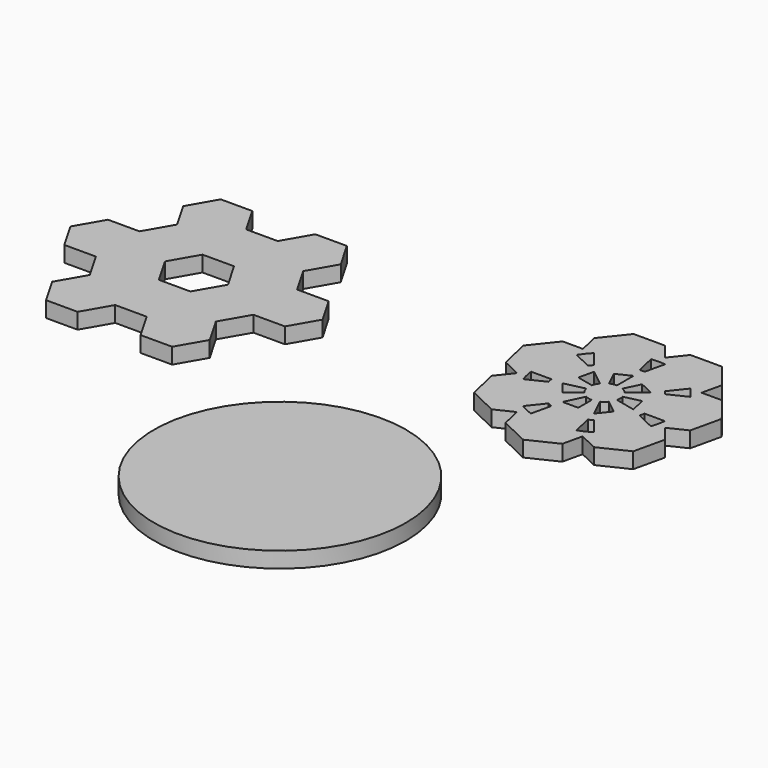
from build123d import *

# Parameters (mm, degrees)
F1_DEPTH = 5
F0_R     = 40


with BuildPart() as f1:
    # F0 (on Top) → F1 (new body)
    with BuildSketch(Plane.XY):
        Polygon((-6.3519277994, -7.4067961433), (-11.3519277994, 1.2534578946), (-21.3519277994, 1.2534578946), (-26.3519277994, -7.4067961433), (-21.3519277994, -16.0670501811), (-11.3519277994, -16.0670501811), align=None)
        Polygon((-6.3519277994, 9.9137119324), (-11.3519277994, 1.2534578946), (-6.3519277994, -7.4067961433), (3.6480722006, -7.4067961433), (8.6480722006, 1.2534578946), (3.6480722006, 9.9137119324), align=None)
        Polygon((-26.3519277994, -7.4067961433), (-21.3519277994, 1.2534578946), (-26.3519277994, 9.9137119324), (-36.3519277994, 9.9137119324), (-41.3519277994, 1.2534578946), (-36.3519277994, -7.4067961433), align=None)
        Polygon((-11.3519277994, 18.5739659703), (-6.3519277994, 9.9137119324), (3.6480722006, 9.9137119324), (8.6480722006, 18.5739659703), (3.6480722006, 27.2342200081), (-6.3519277994, 27.2342200081), align=None)
        Polygon((3.6480722006, -7.4067961433), (-6.3519277994, -7.4067961433), (-11.3519277994, -16.0670501811), (-6.3519277994, -24.727304219), (3.6480722006, -24.727304219), (8.6480722006, -16.0670501811), align=None)
        Polygon((-36.3519277994, 9.9137119324), (-26.3519277994, 9.9137119324), (-21.3519277994, 18.5739659703), (-26.3519277994, 27.2342200081), (-36.3519277994, 27.2342200081), (-41.3519277994, 18.5739659703), align=None)
        Polygon((-21.3519277994, -16.0670501811), (-26.3519277994, -7.4067961433), (-36.3519277994, -7.4067961433), (-41.3519277994, -16.0670501811), (-36.3519277994, -24.727304219), (-26.3519277994, -24.727304219), align=None)
        Polygon((-21.3519277994, 18.5739659703), (-11.3519277994, 18.5739659703), (-6.3519277994, 27.2342200081), (-11.3519277994, 35.894474046), (-21.3519277994, 35.894474046), (-26.3519277994, 27.2342200081), align=None)
        Polygon((8.6480722006, 18.5739659703), (3.6480722006, 9.9137119324), (8.6480722006, 1.2534578946), (18.6480722006, 1.2534578946), (23.6480722006, 9.9137119324), (18.6480722006, 18.5739659703), align=None)
        Polygon((-41.3519277994, 1.2534578946), (-36.3519277994, 9.9137119324), (-41.3519277994, 18.5739659703), (-51.3519277994, 18.5739659703), (-56.3519277994, 9.9137119324), (-51.3519277994, 1.2534578946), align=None)
        Polygon((-11.3519277994, 35.894474046), (-6.3519277994, 27.2342200081), (3.6480722006, 27.2342200081), (8.6480722006, 35.894474046), (3.6480722006, 44.5547280838), (-6.3519277994, 44.5547280838), align=None)
        Polygon((-36.3519277994, 27.2342200081), (-26.3519277994, 27.2342200081), (-21.3519277994, 35.894474046), (-26.3519277994, 44.5547280838), (-36.3519277994, 44.5547280838), (-41.3519277994, 35.894474046), align=None)
    extrude(amount=F1_DEPTH)


with BuildPart() as f1b:
    # F0 (on Top) → F1, piece 2 (new body)
    with BuildSketch(Plane.XY):
        with BuildLine():
            Line((108.4534161646, 9.1103293915), (107.6647373891, 12.5657568802))
            Line((107.6647373891, 12.5657568802), (102.6647373891, 12.5657568802))
            Line((102.6647373891, 12.5657568802), (97.6647373891, 12.5657568802))
            Line((97.6647373891, 12.5657568802), (96.8760586136, 9.1103293915))
            ThreePointArc((96.8760586136, 9.1103293915), (102.6647373891, 7.948363863), (108.4534161646, 9.1103293915))
        make_face()
        with BuildLine():
            Line((109.8745662116, 9.7947191837), (107.6647373891, 12.5657568802))
            Line((107.6647373891, 12.5657568802), (108.4534161646, 9.1103293915))
            ThreePointArc((108.4534161646, 9.1103293915), (109.1729934758, 9.4338308445), (109.8745662116, 9.7947191837))
        make_face()
        with BuildLine():
            Line((110.7821863984, 16.4749142925), (107.6647373891, 12.5657568802))
            Line((107.6647373891, 12.5657568802), (109.8745662116, 9.7947191837))
            ThreePointArc((109.8745662116, 9.7947191837), (114.3922096261, 13.5960168351), (117.0929305771, 18.8462618009))
            Line((117.0929305771, 18.8462618009), (113.8996354077, 20.3840717048))
            Line((113.8996354077, 20.3840717048), (110.7821863984, 16.4749142925))
        make_face()
        with BuildLine():
            Line((102.6647373891, 12.5657568802), (107.6647373891, 12.5657568802))
            Line((107.6647373891, 12.5657568802), (104.8341560847, 18.4435195235))
            ThreePointArc((104.8341560847, 18.4435195235), (103.7773420588, 18.0737243021), (102.6647373891, 17.948363863))
            Line((102.6647373891, 17.948363863), (102.6647373891, 12.5657568802))
        make_face()
        with BuildLine():
            Line((106.5738948014, 19.8309148537), (110.7821863984, 16.4749142925))
            Line((110.7821863984, 16.4749142925), (113.8996354077, 20.3840717048))
            Line((113.8996354077, 20.3840717048), (107.53937695, 21.8357591932))
            ThreePointArc((107.53937695, 21.8357591932), (107.1695817286, 20.7789451674), (106.5738948014, 19.8309148537))
        make_face()
        with BuildLine():
            Line((109.8899467286, 2.8164777583), (108.4534161646, 9.1103293915))
            ThreePointArc((108.4534161646, 9.1103293915), (102.6647373891, 7.948363863), (96.8760586136, 9.1103293915))
            Line((96.8760586136, 9.1103293915), (95.4395280495, 2.8164777583))
            ThreePointArc((95.4395280495, 2.8164777583), (102.6647373891, 1.5591963212), (109.8899467286, 2.8164777583))
        make_face()
        with BuildLine():
            ThreePointArc((117.0929305771, 18.8462618009), (114.3922096261, 13.5960168351), (109.8745662116, 9.7947191837))
            Line((109.8745662116, 9.7947191837), (113.8996354077, 4.7474420555))
            ThreePointArc((113.8996354077, 4.7474420555), (119.3874619571, 9.6124360304), (122.9093240867, 16.0452343137))
            Line((122.9093240867, 16.0452343137), (117.0929305771, 18.8462618009))
        make_face()
        with BuildLine():
            ThreePointArc((102.6647373891, 17.948363863), (103.7773420588, 18.0737243021), (104.8341560847, 18.4435195235))
            Line((104.8341560847, 18.4435195235), (102.6647373891, 22.948363863))
            Line((102.6647373891, 22.948363863), (102.6647373891, 17.948363863))
        make_face()
        with BuildLine():
            Line((102.6647373891, 22.948363863), (104.8341560847, 18.4435195235))
            ThreePointArc((104.8341560847, 18.4435195235), (105.7821863984, 19.0392064507), (106.5738948014, 19.8309148537))
            Line((106.5738948014, 19.8309148537), (102.6647373891, 22.948363863))
        make_face()
        with BuildLine():
            Line((95.4549085665, 9.7947191837), (97.6647373891, 12.5657568802))
            Line((97.6647373891, 12.5657568802), (94.5472883798, 16.4749142925))
            Line((94.5472883798, 16.4749142925), (91.4298393705, 20.3840717048))
            Line((91.4298393705, 20.3840717048), (88.236544201, 18.8462618009))
            ThreePointArc((88.236544201, 18.8462618009), (90.937265152, 13.5960168351), (95.4549085665, 9.7947191837))
        make_face()
        with BuildLine():
            Line((96.8760586136, 9.1103293915), (97.6647373891, 12.5657568802))
            Line((97.6647373891, 12.5657568802), (95.4549085665, 9.7947191837))
            ThreePointArc((95.4549085665, 9.7947191837), (96.1564813023, 9.4338308445), (96.8760586136, 9.1103293915))
        make_face()
        with BuildLine():
            Line((94.5472883798, 16.4749142925), (97.6647373891, 12.5657568802))
            Line((97.6647373891, 12.5657568802), (100.4953186935, 18.4435195235))
            ThreePointArc((100.4953186935, 18.4435195235), (99.5472883798, 19.0392064507), (98.7555799767, 19.8309148537))
            Line((98.7555799767, 19.8309148537), (94.5472883798, 16.4749142925))
        make_face()
        with BuildLine():
            ThreePointArc((100.4953186935, 18.4435195235), (101.5521327193, 18.0737243021), (102.6647373891, 17.948363863))
            Line((102.6647373891, 17.948363863), (102.6647373891, 22.948363863))
            Line((102.6647373891, 22.948363863), (100.4953186935, 18.4435195235))
        make_face()
        with BuildLine():
            Line((117.4439256526, 20.3840717048), (113.8996354077, 20.3840717048))
            Line((113.8996354077, 20.3840717048), (117.0929305771, 18.8462618009))
            ThreePointArc((117.0929305771, 18.8462618009), (117.2886560718, 19.6105498537), (117.4439256526, 20.3840717048))
        make_face()
        with BuildLine():
            Line((112.7870307379, 25.2587112658), (113.8996354077, 20.3840717048))
            Line((113.8996354077, 20.3840717048), (117.4439256526, 20.3840717048))
            ThreePointArc((117.4439256526, 20.3840717048), (117.6094325006, 21.661473027), (117.6647373891, 22.948363863))
            ThreePointArc((117.6647373891, 22.948363863), (116.9483776416, 27.5284971729), (114.8677212376, 31.6711607306))
            Line((114.8677212376, 31.6711607306), (111.6744260681, 30.1333508267))
            Line((111.6744260681, 30.1333508267), (112.7870307379, 25.2587112658))
        make_face()
        with BuildLine():
            Line((102.6647373891, 22.948363863), (106.5738948014, 19.8309148537))
            ThreePointArc((106.5738948014, 19.8309148537), (107.1695817286, 20.7789451674), (107.53937695, 21.8357591932))
            Line((107.53937695, 21.8357591932), (102.6647373891, 22.948363863))
        make_face()
        with BuildLine():
            ThreePointArc((113.8996354077, 4.7474420555), (111.9451493787, 3.6773897975), (109.8899467286, 2.8164777583))
            Line((109.8899467286, 2.8164777583), (113.1054673892, 1.267964622))
            Line((113.1054673892, 1.267964622), (113.8996354077, 4.7474420555))
        make_face()
        with BuildLine():
            Line((113.1054673892, 1.267964622), (109.8899467286, 2.8164777583))
            ThreePointArc((109.8899467286, 2.8164777583), (102.6647373891, 1.5591963212), (95.4395280495, 2.8164777583))
            Line((95.4395280495, 2.8164777583), (92.224007389, 1.267964622))
            Line((92.224007389, 1.267964622), (93.65504871, -5.0018370663))
            ThreePointArc((93.65504871, -5.0018370663), (102.6647373891, -6.4180833529), (111.6744260681, -5.0018370663))
            Line((111.6744260681, -5.0018370663), (113.1054673892, 1.267964622))
        make_face()
        with BuildLine():
            ThreePointArc((122.9093240867, 16.0452343137), (119.3874619571, 9.6124360304), (113.8996354077, 4.7474420555))
            Line((113.8996354077, 4.7474420555), (113.1054673892, 1.267964622))
            Line((113.1054673892, 1.267964622), (118.8996354077, -1.5223596328))
            ThreePointArc((118.8996354077, -1.5223596328), (125.6243503507, 4.6386835071), (130.1345334262, 12.5657568802))
            Line((130.1345334262, 12.5657568802), (126.1248447472, 17.59374745))
            Line((126.1248447472, 17.59374745), (122.9093240867, 16.0452343137))
        make_face()
        with BuildLine():
            Line((97.7900978282, 24.0609685328), (102.6647373891, 22.948363863))
            Line((102.6647373891, 22.948363863), (98.7555799767, 26.0658128723))
            ThreePointArc((98.7555799767, 26.0658128723), (98.1598930496, 25.1177825586), (97.7900978282, 24.0609685328))
        make_face()
        with BuildLine():
            Line((98.7555799767, 26.0658128723), (102.6647373891, 22.948363863))
            Line((102.6647373891, 22.948363863), (100.4953186935, 27.4532082025))
            ThreePointArc((100.4953186935, 27.4532082025), (99.5472883798, 26.8575212754), (98.7555799767, 26.0658128723))
        make_face()
        with BuildLine():
            Line((98.7555799767, 19.8309148537), (102.6647373891, 22.948363863))
            Line((102.6647373891, 22.948363863), (97.7900978282, 21.8357591932))
            ThreePointArc((97.7900978282, 21.8357591932), (98.1598930496, 20.7789451674), (98.7555799767, 19.8309148537))
        make_face()
        with BuildLine():
            Line((106.5738948014, 26.0658128723), (102.6647373891, 22.948363863))
            Line((102.6647373891, 22.948363863), (107.53937695, 24.0609685328))
            ThreePointArc((107.53937695, 24.0609685328), (107.1695817286, 25.1177825586), (106.5738948014, 26.0658128723))
        make_face()
        with BuildLine():
            Line((102.6647373891, 27.948363863), (102.6647373891, 22.948363863))
            Line((102.6647373891, 22.948363863), (104.8341560847, 27.4532082025))
            ThreePointArc((104.8341560847, 27.4532082025), (103.7773420588, 27.8230034239), (102.6647373891, 27.948363863))
        make_face()
        with BuildLine():
            Line((104.8341560847, 27.4532082025), (102.6647373891, 22.948363863))
            Line((102.6647373891, 22.948363863), (106.5738948014, 26.0658128723))
            ThreePointArc((106.5738948014, 26.0658128723), (105.7821863984, 26.8575212754), (104.8341560847, 27.4532082025))
        make_face()
        with BuildLine():
            Line((100.4953186935, 18.4435195235), (102.6647373891, 22.948363863))
            Line((102.6647373891, 22.948363863), (98.7555799767, 19.8309148537))
            ThreePointArc((98.7555799767, 19.8309148537), (99.5472883798, 19.0392064507), (100.4953186935, 18.4435195235))
        make_face()
        with BuildLine():
            Line((107.53937695, 24.0609685328), (102.6647373891, 22.948363863))
            Line((102.6647373891, 22.948363863), (107.53937695, 21.8357591932))
            ThreePointArc((107.53937695, 21.8357591932), (107.6332984385, 22.3885414825), (107.6647373891, 22.948363863))
            ThreePointArc((107.6647373891, 22.948363863), (107.6332984385, 23.5081862435), (107.53937695, 24.0609685328))
        make_face()
        with BuildLine():
            Line((97.7900978282, 21.8357591932), (102.6647373891, 22.948363863))
            Line((102.6647373891, 22.948363863), (97.7900978282, 24.0609685328))
            ThreePointArc((97.7900978282, 24.0609685328), (97.6647373891, 22.948363863), (97.7900978282, 21.8357591932))
        make_face()
        with BuildLine():
            Line((100.4953186935, 27.4532082025), (102.6647373891, 22.948363863))
            Line((102.6647373891, 22.948363863), (102.6647373891, 27.948363863))
            ThreePointArc((102.6647373891, 27.948363863), (101.5521327193, 27.8230034239), (100.4953186935, 27.4532082025))
        make_face()
        with BuildLine():
            Line((91.4298393705, 4.7474420555), (95.4549085665, 9.7947191837))
            ThreePointArc((95.4549085665, 9.7947191837), (90.937265152, 13.5960168351), (88.236544201, 18.8462618009))
            Line((88.236544201, 18.8462618009), (82.4201506915, 16.0452343137))
            ThreePointArc((82.4201506915, 16.0452343137), (85.9420128211, 9.6124360304), (91.4298393705, 4.7474420555))
        make_face()
        with BuildLine():
            Line((107.53937695, 24.0609685328), (112.7870307379, 25.2587112658))
            Line((112.7870307379, 25.2587112658), (111.6744260681, 30.1333508267))
            Line((111.6744260681, 30.1333508267), (106.5738948014, 26.0658128723))
            ThreePointArc((106.5738948014, 26.0658128723), (107.1695817286, 25.1177825586), (107.53937695, 24.0609685328))
        make_face()
        with BuildLine():
            ThreePointArc((117.6647373891, 22.948363863), (117.6094325006, 21.661473027), (117.4439256526, 20.3840717048))
            Line((117.4439256526, 20.3840717048), (123.8996354077, 20.3840717048))
            ThreePointArc((123.8996354077, 20.3840717048), (124.0153027163, 21.6638996403), (124.0539049309, 22.948363863))
            ThreePointArc((124.0539049309, 22.948363863), (123.194179289, 28.9515716231), (120.6841147471, 34.4721882178))
            Line((120.6841147471, 34.4721882178), (114.8677212376, 31.6711607306))
            ThreePointArc((114.8677212376, 31.6711607306), (116.9483776416, 27.5284971729), (117.6647373891, 22.948363863))
        make_face()
        with BuildLine():
            Line((92.224007389, 1.267964622), (95.4395280495, 2.8164777583))
            ThreePointArc((95.4395280495, 2.8164777583), (93.3843253994, 3.6773897975), (91.4298393705, 4.7474420555))
            Line((91.4298393705, 4.7474420555), (92.224007389, 1.267964622))
        make_face()
        with BuildLine():
            ThreePointArc((123.8996354077, 20.3840717048), (123.5176338439, 18.1888263251), (122.9093240867, 16.0452343137))
            Line((122.9093240867, 16.0452343137), (126.1248447472, 17.59374745))
            Line((126.1248447472, 17.59374745), (123.8996354077, 20.3840717048))
        make_face()
        with BuildLine():
            Line((93.65504871, 30.1333508267), (98.7555799767, 26.0658128723))
            ThreePointArc((98.7555799767, 26.0658128723), (99.5472883798, 26.8575212754), (100.4953186935, 27.4532082025))
            Line((100.4953186935, 27.4532082025), (98.1598930496, 32.3027695223))
            Line((98.1598930496, 32.3027695223), (93.65504871, 30.1333508267))
        make_face()
        with BuildLine():
            Line((91.4298393705, 20.3840717048), (97.7900978282, 21.8357591932))
            ThreePointArc((97.7900978282, 21.8357591932), (97.6647373891, 22.948363863), (97.7900978282, 24.0609685328))
            Line((97.7900978282, 24.0609685328), (92.5424440403, 25.2587112658))
            Line((92.5424440403, 25.2587112658), (91.4298393705, 20.3840717048))
        make_face()
        with BuildLine():
            ThreePointArc((102.6647373891, 27.948363863), (103.7773420588, 27.8230034239), (104.8341560847, 27.4532082025))
            Line((104.8341560847, 27.4532082025), (107.1695817286, 32.3027695223))
            Line((107.1695817286, 32.3027695223), (102.6647373891, 34.4721882178))
            Line((102.6647373891, 34.4721882178), (102.6647373891, 27.948363863))
        make_face()
        with BuildLine():
            Line((87.8855491256, 20.3840717048), (91.4298393705, 20.3840717048))
            Line((91.4298393705, 20.3840717048), (92.5424440403, 25.2587112658))
            Line((92.5424440403, 25.2587112658), (93.65504871, 30.1333508267))
            Line((93.65504871, 30.1333508267), (90.4617535406, 31.6711607306))
            ThreePointArc((90.4617535406, 31.6711607306), (88.0408187063, 26.2861778724), (87.8855491256, 20.3840717048))
        make_face()
        with BuildLine():
            Line((88.236544201, 18.8462618009), (91.4298393705, 20.3840717048))
            Line((91.4298393705, 20.3840717048), (87.8855491256, 20.3840717048))
            ThreePointArc((87.8855491256, 20.3840717048), (88.0408187063, 19.6105498537), (88.236544201, 18.8462618009))
        make_face()
        with BuildLine():
            Line((92.224007389, 1.267964622), (91.4298393705, 4.7474420555))
            ThreePointArc((91.4298393705, 4.7474420555), (85.9420128211, 9.6124360304), (82.4201506915, 16.0452343137))
            Line((82.4201506915, 16.0452343137), (79.2046300309, 17.59374745))
            Line((79.2046300309, 17.59374745), (75.1949413519, 12.5657568802))
            ThreePointArc((75.1949413519, 12.5657568802), (79.7051244274, 4.6386835071), (86.4298393705, -1.5223596328))
            Line((86.4298393705, -1.5223596328), (92.224007389, 1.267964622))
        make_face()
        with BuildLine():
            Line((113.8842548906, 32.9043885231), (111.6744260681, 30.1333508267))
            Line((111.6744260681, 30.1333508267), (114.8677212376, 31.6711607306))
            ThreePointArc((114.8677212376, 31.6711607306), (114.3922096261, 32.3007108909), (113.8842548906, 32.9043885231))
        make_face()
        with BuildLine():
            Line((107.1695817286, 32.3027695223), (111.6744260681, 30.1333508267))
            Line((111.6744260681, 30.1333508267), (113.8842548906, 32.9043885231))
            ThreePointArc((113.8842548906, 32.9043885231), (109.1729934758, 36.4628968816), (103.4534161646, 37.9276157065))
            Line((103.4534161646, 37.9276157065), (102.6647373891, 34.4721882178))
            Line((102.6647373891, 34.4721882178), (107.1695817286, 32.3027695223))
        make_face()
        with BuildLine():
            ThreePointArc((124.0539049309, 22.948363863), (124.0153027163, 21.6638996403), (123.8996354077, 20.3840717048))
            Line((123.8996354077, 20.3840717048), (126.1248447472, 17.59374745))
            Line((126.1248447472, 17.59374745), (131.9190127657, 20.3840717048))
            ThreePointArc((131.9190127657, 20.3840717048), (132.0031282428, 21.6649916651), (132.031184605, 22.948363863))
            ThreePointArc((132.031184605, 22.948363863), (130.9819763508, 30.7279653741), (127.9093240867, 37.9516656513))
            Line((127.9093240867, 37.9516656513), (121.4782827656, 37.9516656513))
            Line((121.4782827656, 37.9516656513), (120.6841147471, 34.4721882178))
            ThreePointArc((120.6841147471, 34.4721882178), (123.194179289, 28.9515716231), (124.0539049309, 22.948363863))
        make_face()
        with BuildLine():
            ThreePointArc((130.1345334262, 12.5657568802), (125.6243503507, 4.6386835071), (118.8996354077, -1.5223596328))
            Line((118.8996354077, -1.5223596328), (127.9093240867, 2.8164777583))
            Line((127.9093240867, 2.8164777583), (130.1345334262, 12.5657568802))
        make_face()
        with BuildLine():
            Line((102.6647373891, -9.3406744575), (111.6744260681, -5.0018370663))
            ThreePointArc((111.6744260681, -5.0018370663), (102.6647373891, -6.4180833529), (93.65504871, -5.0018370663))
            Line((93.65504871, -5.0018370663), (102.6647373891, -9.3406744575))
        make_face()
        with BuildLine():
            Line((91.4452198875, 32.9043885231), (93.65504871, 30.1333508267))
            Line((93.65504871, 30.1333508267), (98.1598930496, 32.3027695223))
            Line((98.1598930496, 32.3027695223), (102.6647373891, 34.4721882178))
            Line((102.6647373891, 34.4721882178), (101.8760586136, 37.9276157065))
            ThreePointArc((101.8760586136, 37.9276157065), (96.1564813023, 36.4628968816), (91.4452198875, 32.9043885231))
        make_face()
        with BuildLine():
            Line((90.4617535406, 31.6711607306), (93.65504871, 30.1333508267))
            Line((93.65504871, 30.1333508267), (91.4452198875, 32.9043885231))
            ThreePointArc((91.4452198875, 32.9043885231), (90.937265152, 32.3007108909), (90.4617535406, 31.6711607306))
        make_face()
        with BuildLine():
            Line((101.8760586136, 37.9276157065), (102.6647373891, 34.4721882178))
            Line((102.6647373891, 34.4721882178), (103.4534161646, 37.9276157065))
            ThreePointArc((103.4534161646, 37.9276157065), (102.6647373891, 37.948363863), (101.8760586136, 37.9276157065))
        make_face()
        with BuildLine():
            Line((81.4298393705, 20.3840717048), (87.8855491256, 20.3840717048))
            ThreePointArc((87.8855491256, 20.3840717048), (88.0408187063, 26.2861778724), (90.4617535406, 31.6711607306))
            Line((90.4617535406, 31.6711607306), (84.645360031, 34.4721882178))
            ThreePointArc((84.645360031, 34.4721882178), (81.8118409342, 27.707901401), (81.4298393705, 20.3840717048))
        make_face()
        with BuildLine():
            Line((79.2046300309, 17.59374745), (82.4201506915, 16.0452343137))
            ThreePointArc((82.4201506915, 16.0452343137), (81.8118409342, 18.1888263251), (81.4298393705, 20.3840717048))
            Line((81.4298393705, 20.3840717048), (79.2046300309, 17.59374745))
        make_face()
        with BuildLine():
            ThreePointArc((103.4534161646, 37.9276157065), (109.1729934758, 36.4628968816), (113.8842548906, 32.9043885231))
            Line((113.8842548906, 32.9043885231), (117.9093240867, 37.9516656513))
            ThreePointArc((117.9093240867, 37.9516656513), (111.9451493787, 42.2193379286), (104.8899467286, 44.2214673397))
            Line((104.8899467286, 44.2214673397), (103.4534161646, 37.9276157065))
        make_face()
        with BuildLine():
            Line((77.4201506915, 2.8164777583), (86.4298393705, -1.5223596328))
            ThreePointArc((86.4298393705, -1.5223596328), (79.7051244274, 4.6386835071), (75.1949413519, 12.5657568802))
            Line((75.1949413519, 12.5657568802), (77.4201506915, 2.8164777583))
        make_face()
        with BuildLine():
            ThreePointArc((132.031184605, 22.948363863), (132.0031282428, 21.6649916651), (131.9190127657, 20.3840717048))
            Line((131.9190127657, 20.3840717048), (134.1442221053, 30.1333508267))
            Line((134.1442221053, 30.1333508267), (127.9093240867, 37.9516656513))
            ThreePointArc((127.9093240867, 37.9516656513), (130.9819763508, 30.7279653741), (132.031184605, 22.948363863))
        make_face()
        with BuildLine():
            Line((87.4201506915, 37.9516656513), (91.4452198875, 32.9043885231))
            ThreePointArc((91.4452198875, 32.9043885231), (96.1564813023, 36.4628968816), (101.8760586136, 37.9276157065))
            Line((101.8760586136, 37.9276157065), (100.4395280495, 44.2214673397))
            ThreePointArc((100.4395280495, 44.2214673397), (93.3843253994, 42.2193379286), (87.4201506915, 37.9516656513))
        make_face()
        with BuildLine():
            Line((79.2046300309, 17.59374745), (81.4298393705, 20.3840717048))
            ThreePointArc((81.4298393705, 20.3840717048), (81.8118409342, 27.707901401), (84.645360031, 34.4721882178))
            Line((84.645360031, 34.4721882178), (83.8511920125, 37.9516656513))
            Line((83.8511920125, 37.9516656513), (77.4201506915, 37.9516656513))
            ThreePointArc((77.4201506915, 37.9516656513), (74.0345683167, 29.4830131245), (73.4104620124, 20.3840717048))
            Line((73.4104620124, 20.3840717048), (79.2046300309, 17.59374745))
        make_face()
        with BuildLine():
            ThreePointArc((117.9093240867, 37.9516656513), (119.3874619571, 36.2842916956), (120.6841147471, 34.4721882178))
            Line((120.6841147471, 34.4721882178), (121.4782827656, 37.9516656513))
            Line((121.4782827656, 37.9516656513), (117.9093240867, 37.9516656513))
        make_face()
        with BuildLine():
            ThreePointArc((104.8899467286, 44.2214673397), (111.9451493787, 42.2193379286), (117.9093240867, 37.9516656513))
            Line((117.9093240867, 37.9516656513), (121.4782827656, 37.9516656513))
            Line((121.4782827656, 37.9516656513), (122.9093240867, 44.2214673397))
            ThreePointArc((122.9093240867, 44.2214673397), (115.4063613117, 49.4066185655), (106.6744260681, 52.0397821643))
            Line((106.6744260681, 52.0397821643), (102.6647373891, 47.0117915945))
            Line((102.6647373891, 47.0117915945), (104.8899467286, 44.2214673397))
        make_face()
        with BuildLine():
            Line((83.8511920125, 37.9516656513), (84.645360031, 34.4721882178))
            ThreePointArc((84.645360031, 34.4721882178), (85.9420128211, 36.2842916956), (87.4201506915, 37.9516656513))
            Line((87.4201506915, 37.9516656513), (83.8511920125, 37.9516656513))
        make_face()
        with BuildLine():
            Line((83.8511920125, 37.9516656513), (87.4201506915, 37.9516656513))
            ThreePointArc((87.4201506915, 37.9516656513), (93.3843253994, 42.2193379286), (100.4395280495, 44.2214673397))
            Line((100.4395280495, 44.2214673397), (102.6647373891, 47.0117915945))
            Line((102.6647373891, 47.0117915945), (98.65504871, 52.0397821643))
            ThreePointArc((98.65504871, 52.0397821643), (89.9231134664, 49.4066185655), (82.4201506915, 44.2214673397))
            Line((82.4201506915, 44.2214673397), (83.8511920125, 37.9516656513))
        make_face()
        with BuildLine():
            Line((102.6647373891, 47.0117915945), (100.4395280495, 44.2214673397))
            ThreePointArc((100.4395280495, 44.2214673397), (102.6647373891, 44.3375314049), (104.8899467286, 44.2214673397))
            Line((104.8899467286, 44.2214673397), (102.6647373891, 47.0117915945))
        make_face()
        with BuildLine():
            Line((71.1852526729, 30.1333508267), (73.4104620124, 20.3840717048))
            ThreePointArc((73.4104620124, 20.3840717048), (74.0345683167, 29.4830131245), (77.4201506915, 37.9516656513))
            Line((77.4201506915, 37.9516656513), (71.1852526729, 30.1333508267))
        make_face()
        with BuildLine():
            ThreePointArc((106.6744260681, 52.0397821643), (115.4063613117, 49.4066185655), (122.9093240867, 44.2214673397))
            Line((122.9093240867, 44.2214673397), (116.6744260681, 52.0397821643))
            Line((116.6744260681, 52.0397821643), (106.6744260681, 52.0397821643))
        make_face()
        with BuildLine():
            Line((88.65504871, 52.0397821643), (82.4201506915, 44.2214673397))
            ThreePointArc((82.4201506915, 44.2214673397), (89.9231134664, 49.4066185655), (98.65504871, 52.0397821643))
            Line((98.65504871, 52.0397821643), (88.65504871, 52.0397821643))
        make_face()
    extrude(amount=F1_DEPTH)


with BuildPart() as f1c:
    # F0 (on Top) → F1, piece 3 (new body)
    with BuildSketch(Plane.XY):
        with Locations((67.9241418839, -62.2974261642)):
            Circle(F0_R)
    extrude(amount=F1_DEPTH)


solid = Compound([f1.part, f1b.part, f1c.part])
